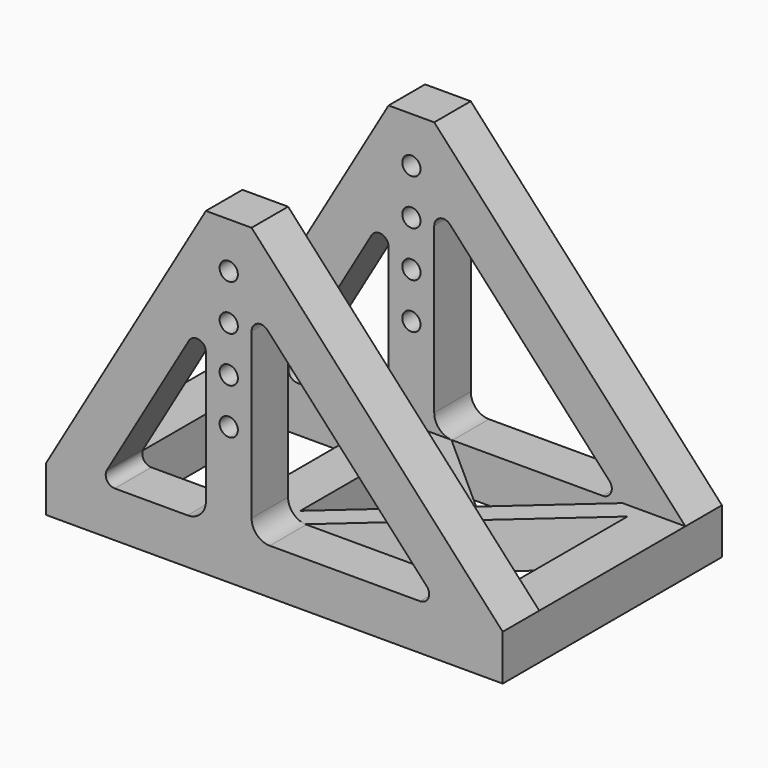
from build123d import *

# Parameters (mm, degrees)
F0_R        = 2.2479
F1_DEPTH    = 76.2
F2_W        = 50.8
F2_H        = 76.2
F3_DEPTH    = 254
F5_DEPTH    = 25.4
F6_T1_DEPTH = 12.7
F6_T3_DEPTH = 12.7
F7_T1_DEPTH = 12.7
F7_T3_DEPTH = 12.7
F8_R        = 2.54
F9_R        = 2.54
F10_DEPTH   = 254


# Not quite as in the source:
# - a fillet or chamfer that OpenCascade refuses, or shapes differently, is made with other operations: its cross-section is extruded or revolved along the edge and cut away or added


with BuildPart() as f1:
    # F0 (on Front) → F1 (new body)
    with BuildSketch(Plane.XZ):
        Polygon((-50.8, 0), (0, 0), (76.2, 0), (76.2, 12.7), (6.35, 88.9), (-6.35, 88.9), (-50.8, 12.7), align=None)
        Polygon((-6.35, 12.7), (-36.0971634445, 12.7), (-6.35, 63.6951373334), align=None, mode=Mode.SUBTRACT)
        with Locations((0, 38.1)):
            Circle(F0_R, mode=Mode.SUBTRACT)
        Polygon((6.35, 12.7), (6.35, 70.1053616754), (58.9715815358, 12.7), align=None, mode=Mode.SUBTRACT)
        with Locations((0, 50.8)):
            Circle(F0_R, mode=Mode.SUBTRACT)
        with Locations((0, 63.5)):
            Circle(F0_R, mode=Mode.SUBTRACT)
        with Locations((0, 76.2)):
            Circle(F0_R, mode=Mode.SUBTRACT)
    extrude(amount=F1_DEPTH)

    # F2 (on face) → F3 (cut)
    with BuildSketch(Plane(origin=(-50.8, 0, 0), x_dir=(0, -1, 0), z_dir=(-1, 0, 0))):
        with Locations((38.1, 50.8)):
            Rectangle(F2_W, F2_H)
    extrude(amount=-F3_DEPTH, mode=Mode.SUBTRACT)

    # F4 (on face) → F5 (cut)
    with BuildSketch(Plane.XY.offset(12.7)):
        Polygon((58.7209921515, -12.7), (11.1290078485, -12.7), (34.925, -33.8519930236), align=None)
        Polygon((34.925, -42.3480069764), (11.1290078485, -63.5), (58.7209921515, -63.5), align=None)
        Polygon((-36.0971634445, -12.7), (-38.1, -12.7), (-38.1, -63.5), (-36.0971634445, -63.5), (-6.35, -63.5), (-6.35, -12.7), align=None)
        Polygon((30.1459921515, -38.1), (6.35, -16.9480069764), (6.35, -59.2519930236), align=None)
        Polygon((63.5, -59.2519930236), (63.5, -16.9480069764), (39.7040078485, -38.1), align=None)
    extrude(amount=-F5_DEPTH, mode=Mode.SUBTRACT)

    # F6: fillet of radius 5.08 on 4 edges, made by hand

    # F6_s2 → F6_t1 (join)
    with BuildSketch(Plane.XZ.offset(63.5)):
        with BuildLine():
            ThreePointArc((-11.43, 12.7), (-7.8378975516, 14.1878975516), (-6.35, 17.78))
            Line((-6.35, 17.78), (-6.35, 12.7))
            Line((-6.35, 12.7), (-11.43, 12.7))
        make_face()
        with BuildLine():
            ThreePointArc((11.43, 12.7), (7.8378975516, 14.1878975516), (6.35, 17.78))
            Line((6.35, 17.78), (6.35, 12.7))
            Line((6.35, 12.7), (11.43, 12.7))
        make_face()
    extrude(amount=F6_T1_DEPTH)

    # F6_s4 → F6_t3 (join)
    with BuildSketch(Plane.XZ):
        with BuildLine():
            ThreePointArc((-11.43, 12.7), (-7.8378975516, 14.1878975516), (-6.35, 17.78))
            Line((-6.35, 17.78), (-6.35, 12.7))
            Line((-6.35, 12.7), (-11.43, 12.7))
        make_face()
        with BuildLine():
            ThreePointArc((11.43, 12.7), (7.8378975516, 14.1878975516), (6.35, 17.78))
            Line((6.35, 17.78), (6.35, 12.7))
            Line((6.35, 12.7), (11.43, 12.7))
        make_face()
    extrude(amount=F6_T3_DEPTH)

    # F7: fillet of radius 2.54 on 7 edges, made by hand

    # F7_s2 → F7_t1 (join)
    with BuildSketch(Plane.XZ.offset(63.5)):
        with BuildLine():
            ThreePointArc((-6.35, 54.2998790858), (-8.2271108528, 56.751853388), (-11.0839984083, 55.5797114907))
            Line((-11.0839984083, 55.5797114907), (-6.35, 63.6951373334))
            Line((-6.35, 63.6951373334), (-6.35, 54.2998790858))
        make_face()
        with BuildLine():
            ThreePointArc((55.0699360257, 16.9563405564), (55.5225489196, 14.2172353676), (53.1975645096, 12.7))
            Line((53.1975645096, 12.7), (58.9715815358, 12.7))
            Line((58.9715815358, 12.7), (55.0699360257, 16.9563405564))
        make_face()
        with BuildLine():
            ThreePointArc((10.7623715161, 65.291865476), (7.9691915647, 65.9427409692), (6.35, 63.5755249196))
            Line((6.35, 63.5755249196), (6.35, 70.1053616754))
            Line((6.35, 70.1053616754), (10.7623715161, 65.291865476))
        make_face()
    extrude(amount=F7_T1_DEPTH)

    # F7_s4 → F7_t3 (join)
    with BuildSketch(Plane.XZ):
        with BuildLine():
            ThreePointArc((6.35, 63.5755249196), (7.9691915647, 65.9427409692), (10.7623715161, 65.291865476))
            Line((10.7623715161, 65.291865476), (6.35, 70.1053616754))
            Line((6.35, 70.1053616754), (6.35, 63.5755249196))
        make_face()
        with BuildLine():
            ThreePointArc((-11.0839984083, 55.5797114907), (-8.2271108528, 56.751853388), (-6.35, 54.2998790858))
            Line((-6.35, 54.2998790858), (-6.35, 63.6951373334))
            Line((-6.35, 63.6951373334), (-11.0839984083, 55.5797114907))
        make_face()
        with BuildLine():
            ThreePointArc((55.0699360257, 16.9563405564), (55.5225489196, 14.2172353676), (53.1975645096, 12.7))
            Line((53.1975645096, 12.7), (58.9715815358, 12.7))
            Line((58.9715815358, 12.7), (55.0699360257, 16.9563405564))
        make_face()
        with BuildLine():
            ThreePointArc((-33.868927875, 16.5198324048), (-33.8774705343, 13.9749257548), (-31.6749294667, 12.7))
            Line((-31.6749294667, 12.7), (-36.0971634445, 12.7))
            Line((-36.0971634445, 12.7), (-33.868927875, 16.5198324048))
        make_face()
    extrude(amount=F7_T3_DEPTH)

    # F8
    f8_edges = [f1.edges().sort_by_distance(p)[0] for p in [
        (-36.097163, -69.85, 12.7),
    ]]
    fillet(f8_edges, radius=F8_R)

    # F9 (on face) → F10 (cut)
    with BuildSketch(Plane.XZ.offset(76.2)):
        with Locations((0, 76.2)):
            Circle(F9_R)
        with Locations((0, 63.5)):
            Circle(F9_R)
        with Locations((0, 50.8)):
            Circle(F9_R)
        with Locations((0, 38.1)):
            Circle(F9_R)
    extrude(amount=-F10_DEPTH, mode=Mode.SUBTRACT)


solid = f1.part
